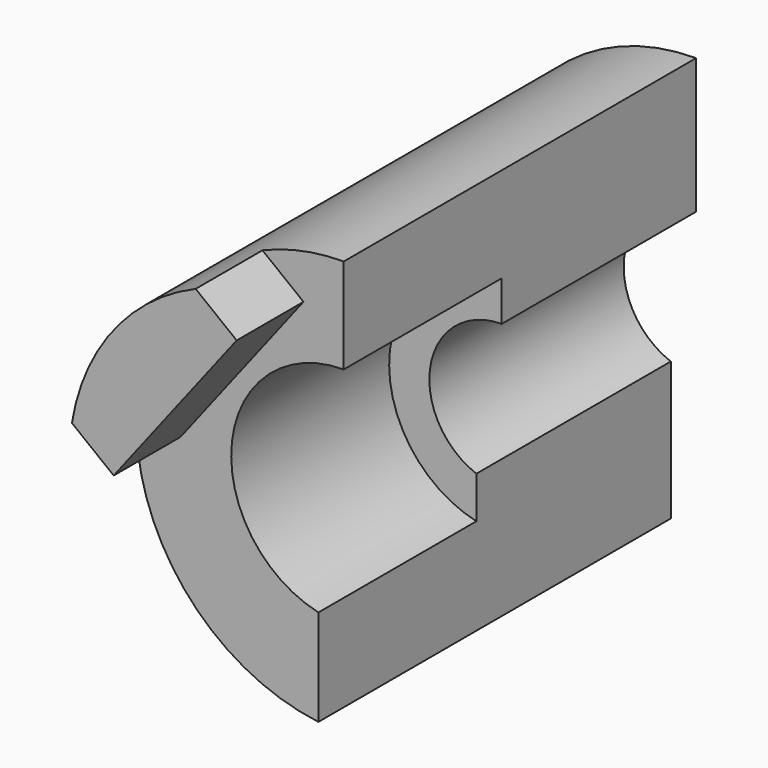
from build123d import *

# Parameters (mm, degrees)
F0_R          = 82
F1_DEPTH      = 25
F1_DEPTH_BACK = 149
F2_R          = 28.575
F3_DEPTH      = 174.001
F6_DEPTH      = 33
F7_R          = 44.45
F7_R_2        = 28.575
F8_DEPTH      = 78
F10_DEPTH     = 174.001


with BuildPart() as f1:
    # F0 (on Front) → F1 (new body, two sides)
    with BuildSketch(Plane.XZ) as f1_sk:
        Circle(F0_R)
    extrude(amount=F1_DEPTH)
    extrude(f1_sk.sketch, amount=-F1_DEPTH_BACK)

    # F2 (on face) → F3 (cut, through all)
    with BuildSketch(Plane.XZ.offset(25)):
        Circle(F2_R)
    extrude(amount=-F3_DEPTH, mode=Mode.SUBTRACT)

    # F4 (on face) → F6 (join)
    with BuildSketch(Plane.XZ.offset(25)):
        with BuildLine():
            ThreePointArc((-32.0991935027, 75.4562242395), (-64.6168817958, 50.4842409767), (-80.9803496399, 12.8911974698))
            Line((-80.9803496399, 12.8911974698), (-64.4803693095, 0))
            Line((-64.4803693095, 0), (-15.8976419198, 62.7981848607))
            Line((-15.8976419198, 62.7981848607), (-32.0991935027, 75.4562242395))
        make_face()
    extrude(amount=F6_DEPTH)

    # F7 (on face) → F8 (cut)
    with BuildSketch(Plane.XZ.offset(25)):
        Circle(F7_R)
        Circle(F7_R_2, mode=Mode.SUBTRACT)
    extrude(amount=-F8_DEPTH, mode=Mode.SUBTRACT)

    # F9 (on face) → F10 (cut, through all)
    with BuildSketch(Plane.XZ.offset(25)):
        with BuildLine():
            Line((91, 95.2523052692), (0, 95.2523052692))
            Line((0, 95.2523052692), (0, 82))
            ThreePointArc((0, 82), (57.9827560573, 57.9827560573), (82, 0))
            ThreePointArc((82, 0), (54.3323108288, -61.4166101311), (-10, -81.3879597975))
            Line((-10, -81.3879597975), (-10, -94.1154360771))
            Line((-10, -94.1154360771), (91, -94.1154360771))
            Line((91, -94.1154360771), (91, 95.2523052692))
        make_face()
        with BuildLine():
            ThreePointArc((82, 0), (57.9827560573, 57.9827560573), (0, 82))
            Line((0, 82), (0, 28.575))
            ThreePointArc((0, 28.575), (20.2055762724, 20.2055762724), (28.575, 0))
            ThreePointArc((28.575, 0), (16.2908045381, -23.4763777551), (-10, -26.7680896778))
            Line((-10, -26.7680896778), (-10, -81.3879597975))
            ThreePointArc((-10, -81.3879597975), (54.3323108288, -61.4166101311), (82, 0))
        make_face()
    extrude(amount=-F10_DEPTH, mode=Mode.SUBTRACT)


solid = f1.part
